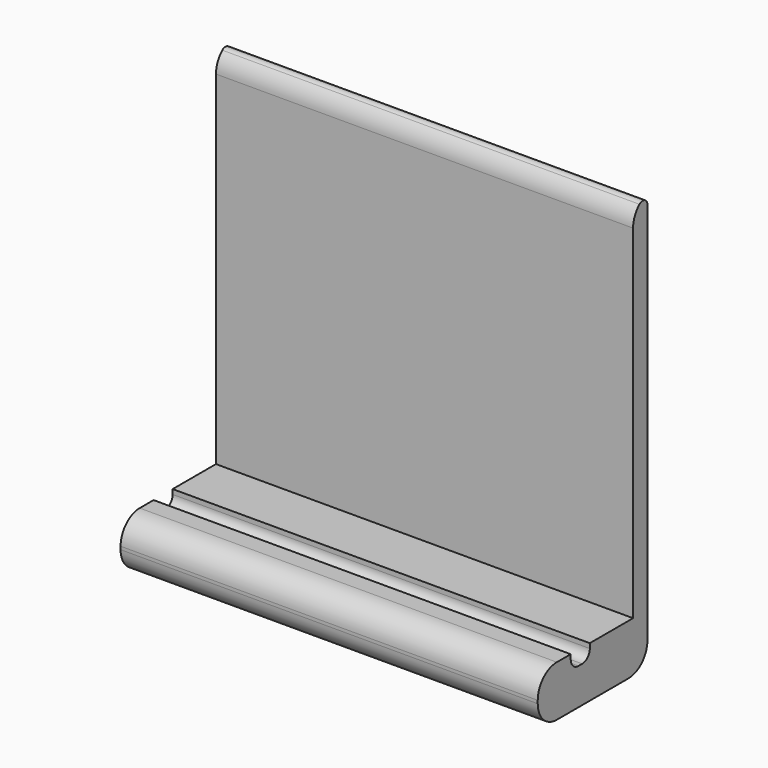
from build123d import *

# Parameters (mm, degrees)
F0_W        = 88.9
F0_H        = 10.8020305634
F1_DEPTH    = 25.4
F3_W        = 88.9
F3_H        = 10.8020305634
F3_H_2      = 78.0979694366
F4_DEPTH    = 3.81
F5_W        = 88.9
F5_H        = 5.08
F6_DEPTH    = 3.048
F7_T1_DEPTH = 113.4934442484
F7_T3_DEPTH = 114.3
F8_R        = 1.27
F9_R        = 2.032


# Not quite as in the source:
# - a fillet or chamfer that OpenCascade refuses, or shapes differently, is made with other operations: its cross-section is extruded or revolved along the edge and cut away or added
# - a feature names something its author has since deleted; it is built from what else it names


with BuildPart() as f1:
    # F0 (on Front) → F1 (new body)
    with BuildSketch(Plane.XZ):
        with Locations((7.6519327545, -42.832814157)):
            Rectangle(F0_W, F0_H)
    extrude(amount=F1_DEPTH)

    # F3 (on face) → F4 (join)
    with BuildSketch(Plane(origin=(0, 0, 0), x_dir=(-1, 0, 0), z_dir=(0, 1, 0))):
        with Locations((-7.6519327545, -42.832814157)):
            Rectangle(F3_W, F3_H)
        with Locations((-7.6519327545, 1.617185843)):
            Rectangle(F3_W, F3_H_2)
    extrude(amount=F4_DEPTH)

    # F5 (on face) → F6 (cut)
    with BuildSketch(Plane.XY.offset(-37.4317988753)):
        with Locations((7.6519327545, -14.0730550206)):
            Rectangle(F5_W, F5_H)
    extrude(amount=-F6_DEPTH, mode=Mode.SUBTRACT)

    # F7: fillet of radius 5.08 on 4 edges, made by hand

    # F7_s2 → F7_t1 (cut)
    with BuildSketch(Plane.YZ.offset(-49.0947893697)):
        with BuildLine():
            ThreePointArc((0, 35.7474817116), (1.0639073716, 38.858333685), (3.81, 40.6661705613))
            Line((3.81, 40.6661705613), (0, 40.6661705613))
            Line((0, 40.6661705613), (0, 35.7474817116))
        make_face()
    extrude(amount=F7_T1_DEPTH, mode=Mode.SUBTRACT)

    # F7_s4 → F7_t3 (cut)
    with BuildSketch(Plane.YZ.offset(-49.4980672455)):
        with BuildLine():
            ThreePointArc((-25.4, -42.5117988753), (-23.9121024484, -38.9196964269), (-20.32, -37.4317988753))
            Line((-20.32, -37.4317988753), (-25.4, -37.4317988753))
            Line((-25.4, -37.4317988753), (-25.4, -42.5117988753))
        make_face()
        with BuildLine():
            ThreePointArc((-20.32, -48.2338294387), (-23.9121024484, -46.7459318871), (-25.4, -43.1538294387))
            Line((-25.4, -43.1538294387), (-25.4, -48.2338294387))
            Line((-25.4, -48.2338294387), (-20.32, -48.2338294387))
        make_face()
        with BuildLine():
            ThreePointArc((3.81, -43.1538294387), (2.3221024484, -46.7459318871), (-1.27, -48.2338294387))
            Line((-1.27, -48.2338294387), (3.81, -48.2338294387))
            Line((3.81, -48.2338294387), (3.81, -43.1538294387))
        make_face()
    extrude(amount=F7_T3_DEPTH, mode=Mode.SUBTRACT)

    # F8
    f8_edges = [f1.edges().sort_by_distance(p)[0] for p in [
        (7.651933, 3.81, 40.666171),
    ]]
    fillet(f8_edges, radius=F8_R)

    # F9
    f9_edges = [f1.edges().sort_by_distance(p)[0] for p in [
        (7.651933, -16.613055, -40.479799),
        (7.651933, -11.533055, -40.479799),
    ]]
    fillet(f9_edges, radius=F9_R)


solid = f1.part
